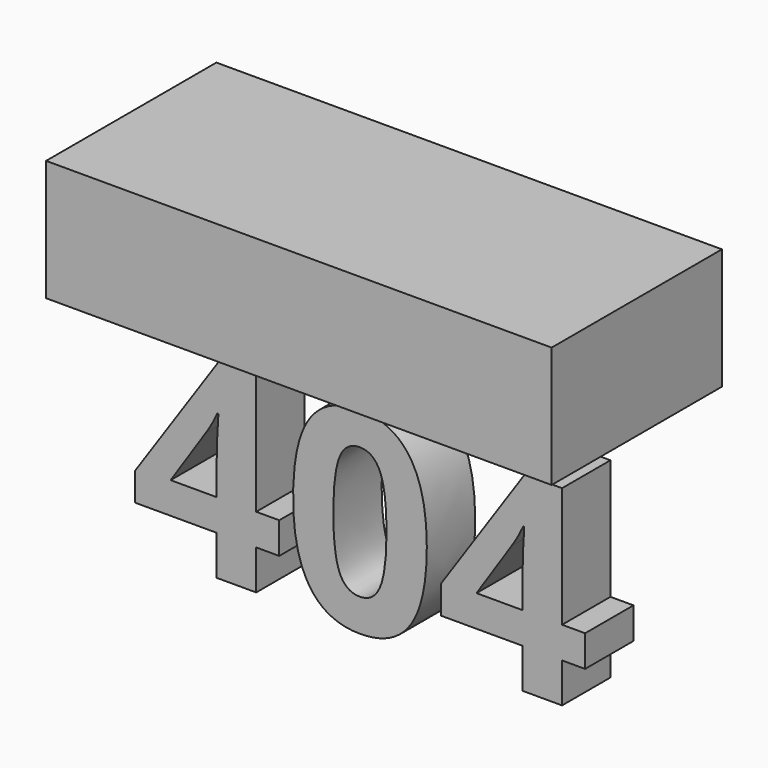
from build123d import *

# Parameters (mm, degrees)
F0_TEXT_SIZE = 56.2680574755
F1_DEPTH     = 12.7
F2_W         = 106.1719991267
F2_H         = 44.7040013969
F3_DEPTH     = 25.4


# Not quite as in the source:
# - Text() gives the source's letters only with a copy of the font that has no kerning and outlines rounded to 1/6400 em; it was checked with that copy


with BuildPart() as f1:
    # F0 (on Front) → F1 (new body)
    with BuildSketch(Plane.XZ):
        with Locations((-63.6270046234, 0)):
            Text('404', F0_TEXT_SIZE, font='Open Sans', font_style=FontStyle.BOLD, text_align=(TextAlign.LEFT, TextAlign.BOTTOM))
    extrude(amount=F1_DEPTH)


with BuildPart() as f3:
    # F2 (on Top) → F3 (new body)
    with BuildSketch(Plane.XY):
        with Locations((-15.3669994324, -6.4770001918)):
            Rectangle(F2_W, F2_H)
    extrude(amount=F3_DEPTH)


with BuildPart() as f3_1:
    # F4: moved
    add(f3.part.moved(Location((0, 0, 50.8))))


solid = Compound([f1.part, f3_1.part])
